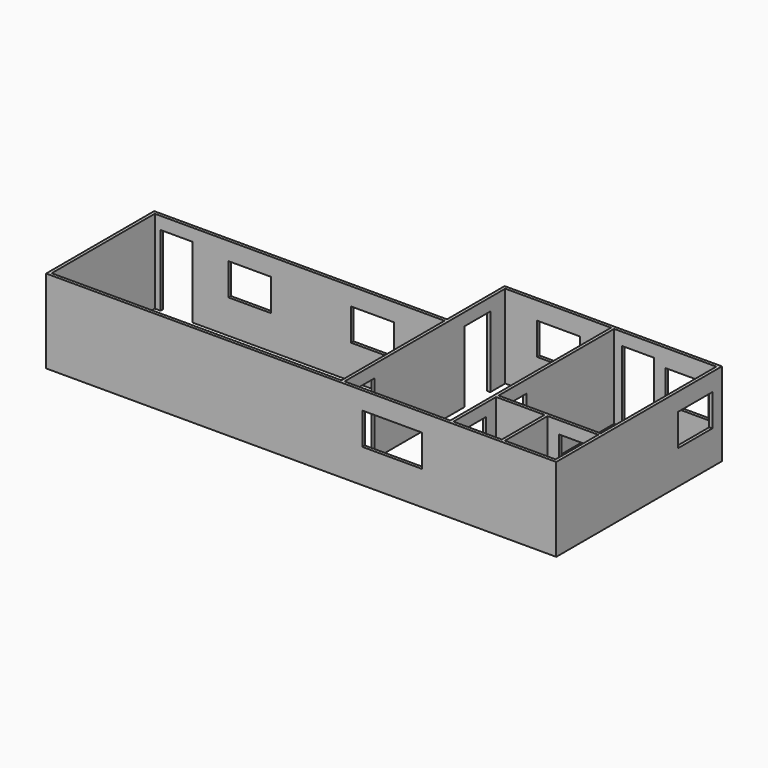
from build123d import *

# Parameters (mm, degrees)
F0_W     = 8280.4
F0_H     = 3683
F0_W_2   = 1384.3
F0_H_2   = 1524
F0_W_3   = 1447.8
F0_W_4   = 3022.6
F0_H_3   = 5740.4
F0_W_5   = 2921
F0_H_4   = 4127.5
F1_DEPTH = 2387.6
F2_W     = 914.4
F2_H     = 88.9
F2_W_2   = 88.9
F2_H_2   = 812.8
F2_H_3   = 914.4
F2_W_3   = 812.8
F3_DEPTH = 2032
F5_W     = 1219.2
F5_H     = 88.9
F5_W_2   = 88.9
F5_H_2   = 1219.2
F5_W_3   = 1701.8
F7_DEPTH = 914.4


# Not quite as in the source:
# - a feature of the source that left no trace in its solid (it failed there, or was rolled back) is left out


with BuildPart() as f1:
    # F0 (on Top) → F1 (new body)
    with BuildSketch(Plane.XY):
        Polygon((0, 3860.8), (0, 0), (14579.6, 0), (14579.6, 5918.2), (8369.3, 5918.2), (8369.3, 3860.8), align=None)
        with Locations((4229.1, 1930.4)):
            Rectangle(F0_W, F0_H, mode=Mode.SUBTRACT)
        with Locations((12261.85, 850.9)):
            Rectangle(F0_W_2, F0_H_2, mode=Mode.SUBTRACT)
        with Locations((13766.8, 850.9)):
            Rectangle(F0_W_3, F0_H_2, mode=Mode.SUBTRACT)
        with Locations((9969.5, 2959.1)):
            Rectangle(F0_W_4, F0_H_3, mode=Mode.SUBTRACT)
        with Locations((13030.2, 3765.55)):
            Rectangle(F0_W_5, F0_H_4, mode=Mode.SUBTRACT)
    extrude(amount=F1_DEPTH)

    # F2 (on Top) → F3 (cut)
    with BuildSketch(Plane.XY):
        with Locations((711.2, 3816.35)):
            Rectangle(F2_W, F2_H)
        with Locations((8413.75, 749.3)):
            Rectangle(F2_W_2, F2_H_2)
        with Locations((8413.75, 4838.7)):
            Rectangle(F2_W_2, F2_H_3)
        with Locations((12255.5, 5873.75)):
            Rectangle(F2_W, F2_H)
        with Locations((11525.25, 850.9)):
            Rectangle(F2_W_2, F2_H_2)
        with Locations((13779.5, 1657.35)):
            Rectangle(F2_W_3, F2_H)
        with Locations((11525.25, 2286)):
            Rectangle(F2_W_2, F2_H_2)
    extrude(amount=F3_DEPTH, mode=Mode.SUBTRACT)

    # F5 (on offset) → F7 (cut, through all)
    with BuildSketch(Plane.XY.offset(965.2)):
        with Locations((2806.7, 3816.35)):
            Rectangle(F5_W, F5_H)
        with Locations((6311.9, 3816.35)):
            Rectangle(F5_W, F5_H)
        with Locations((9982.2, 5873.75)):
            Rectangle(F5_W, F5_H)
        with Locations((13652.5, 5873.75)):
            Rectangle(F5_W, F5_H)
        with Locations((14535.15, 4965.7)):
            Rectangle(F5_W_2, F5_H_2)
        with Locations((9893.3, 44.45)):
            Rectangle(F5_W_3, F5_H)
    extrude(amount=F7_DEPTH, mode=Mode.SUBTRACT)


solid = f1.part
